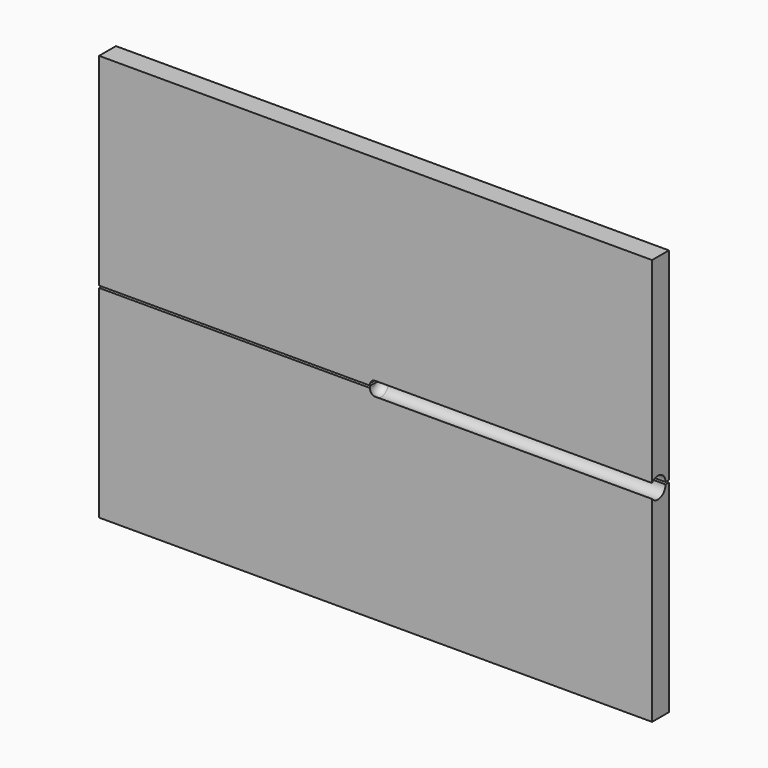
from build123d import *

# Parameters (mm, degrees)
F0_W     = 525
F0_H     = 192
F1_DEPTH = 20
F3_DEPTH = 270
F4_R     = 7


with BuildPart() as f1:
    # F0 (on Front) → F1 (new body)
    with BuildSketch(Plane.XZ):
        with Locations((1.0621380061, 22.721197979)):
            Rectangle(F0_W, F0_H)
    extrude(amount=-F1_DEPTH)

    # F2 (on face) → F3 (cut)
    with BuildSketch(Plane.YZ.offset(263.5621380061)):
        with BuildLine():
            ThreePointArc((0, -67.6219477715), (4, -81.7640833952), (16, -73.278802021))
            Line((16, -73.278802021), (0, -73.278802021))
            Line((0, -73.278802021), (0, -67.6219477715))
        make_face()
        with BuildLine():
            Line((0, -73.278802021), (16, -73.278802021))
            ThreePointArc((16, -73.278802021), (10, -64.7935206468), (0, -67.6219477715))
            Line((0, -67.6219477715), (0, -73.278802021))
        make_face()
    extrude(amount=-F3_DEPTH, mode=Mode.SUBTRACT)

    # F4
    f4_edges = [f1.edges().sort_by_distance(p)[0] for p in [
        (-6.437862, 10, -64.793521),
    ]]
    fillet(f4_edges, radius=F4_R)


with BuildPart() as f7_1:
    # F7: instance of F1
    add(f1.part.mirror(Plane(origin=(-53.484370932, 25, -74.278802021), x_dir=(1, 0, 0), z_dir=(0, 0, 1))))


solid = Compound([f1.part, f7_1.part])
